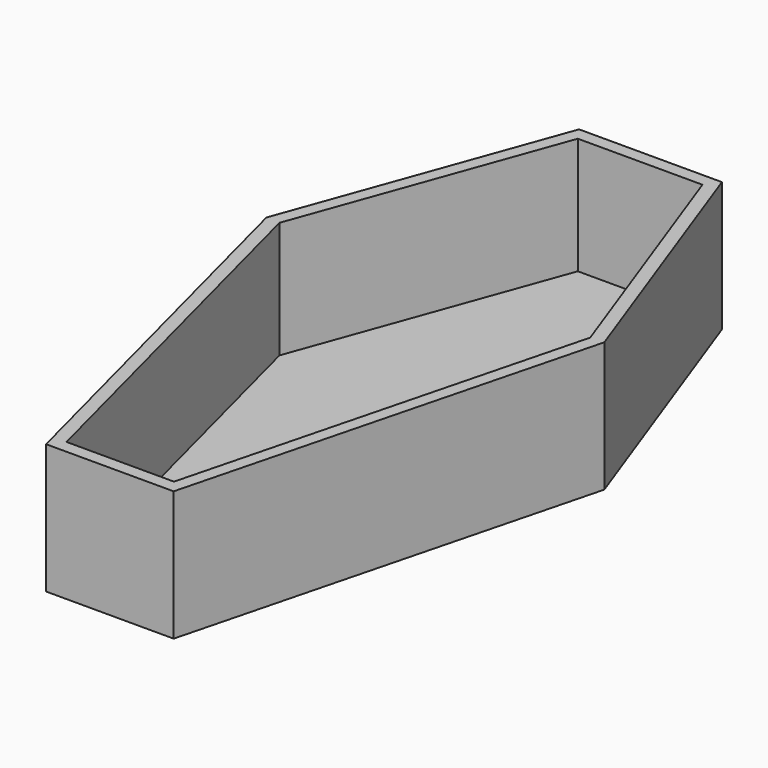
from build123d import *

# Parameters (mm, degrees)
F1_DEPTH = 25.4
F2_T     = -2.54


# Not quite as in the source:
# - a feature of the source that left no trace in its solid (it failed there, or was rolled back) is left out


with BuildPart() as f1:
    # F0 (on Top) → F1 (new body)
    with BuildSketch(Plane.XY):
        Polygon((0, 74.6065601707), (0, -57.7306561172), (12.4910129234, -57.7306561172), (33.0843068659, 21.9417531043), (13.9860804434, 74.6065601707), align=None)
        Polygon((-12.4910129234, -57.7306561172), (0, -57.7306561172), (0, 74.6065601707), (-13.9860804434, 74.6065601707), (-33.0843068659, 21.9417531043), align=None)
    extrude(amount=F1_DEPTH)

    # F2
    f2_openings = [f1.faces().sort_by_distance(p)[0] for p in [
        (0, 11.07211, 25.4),
    ]]
    offset(amount=F2_T, openings=f2_openings)


solid = f1.part
